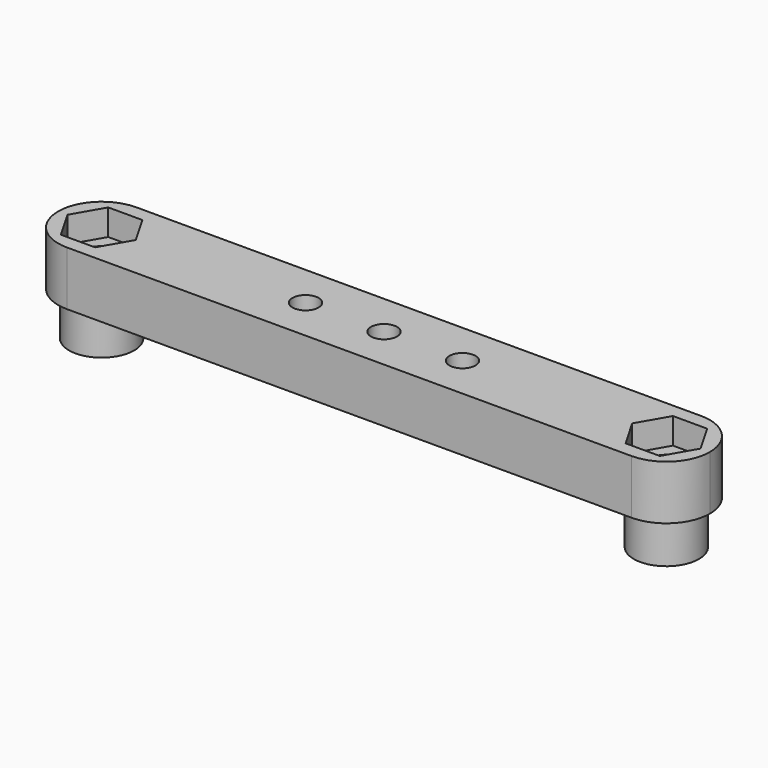
from build123d import *

# Parameters (mm, degrees)
F2_W      = 60
F2_H      = 8
F2_R      = 3
F5_DEPTH  = 5
F1_R      = 3
F1_R_2    = 1.7
F6_DEPTH  = 4
F0_R      = 1.7
F7_DEPTH  = 12.5
F3_R      = 2.05
F8_DEPTH  = 2
F9_DEPTH  = 2
F11_DEPTH = 2.4
F12_R     = 3.99999
F4_R      = 1.2
F13_DEPTH = 5.001


# Not quite as in the source:
# - a fillet or chamfer is up to 0.001 mm smaller than in the source, because OpenCascade refuses the exact size


with BuildPart() as f5:
    # F2 (on face) → F5 (new body)
    with BuildSketch(Plane.XY):
        with Locations((0, 38)):
            Rectangle(F2_W, F2_H)
        with Locations((-26, 38)):
            Circle(F2_R, mode=Mode.SUBTRACT)
        Polygon((1.1402667816, 36.025), (0, 36.025), (-1.1402667816, 36.025), (-2.2805335633, 38), (-1.1402667816, 39.975), (0, 39.975), (1.1402667816, 39.975), (2.2805335633, 38), align=None, mode=Mode.SUBTRACT)
        with Locations((26, 38)):
            Circle(F2_R, mode=Mode.SUBTRACT)
        Polygon((-1.1402667816, 36.025), (0, 36.025), (1.1402667816, 36.025), (2.2805335633, 38), (1.1402667816, 39.975), (0, 39.975), (-1.1402667816, 39.975), (-2.2805335633, 38), align=None)
        with Locations((-26, 38)):
            Circle(F2_R)
        with Locations((26, 38)):
            Circle(F2_R)
    extrude(amount=F5_DEPTH)

    # F1 (on Top) → F6 (join)
    with BuildSketch(Plane.XY):
        with Locations((-26, 38)):
            Circle(F1_R)
        with Locations((-26, 38)):
            Circle(F1_R_2, mode=Mode.SUBTRACT)
        with Locations((26, 38)):
            Circle(F1_R)
        with Locations((26, 38)):
            Circle(F1_R_2, mode=Mode.SUBTRACT)
    extrude(amount=-F6_DEPTH)

    # F0 (on Top) → F7 (cut, symmetric)
    with BuildSketch(Plane.XY):
        with Locations((-26, 38)):
            Circle(F0_R)
        with Locations((26, 38)):
            Circle(F0_R)
        with Locations((-26, -38)):
            Circle(F0_R)
        with Locations((26, -38)):
            Circle(F0_R)
    extrude(amount=F7_DEPTH, both=True, mode=Mode.SUBTRACT)

    # F3 (on face) → F8 (cut)
    with BuildSketch(Plane.XY):
        with Locations((-7.225, 38)):
            Circle(F3_R)
        with Locations((7.225, 38)):
            Circle(F3_R)
    extrude(amount=F8_DEPTH, mode=Mode.SUBTRACT)

    # F2 (on face) → F9 (cut)
    with BuildSketch(Plane.XY):
        Polygon((-1.1402667816, 36.025), (0, 36.025), (1.1402667816, 36.025), (2.2805335633, 38), (1.1402667816, 39.975), (0, 39.975), (-1.1402667816, 39.975), (-2.2805335633, 38), align=None)
    extrude(amount=F9_DEPTH, mode=Mode.SUBTRACT)

    # F10 (on face) → F11 (cut)
    with BuildSketch(Plane.XY.offset(5)):
        Polygon((-27.5732794835, 35.275), (-26, 35.275), (-24.4267205165, 35.275), (-22.8534410329, 38), (-24.4267205165, 40.725), (-26, 40.725), (-27.5732794835, 40.725), (-29.1465589671, 38), align=None)
        Polygon((22.8534410329, 38), (24.4267205165, 35.275), (26, 35.275), (27.5732794835, 35.275), (29.1465589671, 38), (27.5732794835, 40.725), (26, 40.725), (24.4267205165, 40.725), align=None)
    extrude(amount=-F11_DEPTH, mode=Mode.SUBTRACT)

    # F12 (radius 4 in the source; OpenCascade refuses exactly that, so slightly less here)
    f12_edges = [f5.edges().sort_by_distance(p)[0] for p in [
        (-30, 42, 2.5),
        (-30, 34, 2.5),
        (30, 42, 2.5),
        (30, 34, 2.5),
    ]]
    fillet(f12_edges, radius=F12_R)

    # F4 (on face) → F13 (cut, through all)
    with BuildSketch(Plane.XY):
        with Locations((-7.225, 38)):
            Circle(F4_R)
        with Locations((0, 38)):
            Circle(F4_R)
        with Locations((7.225, 38)):
            Circle(F4_R)
    extrude(amount=F13_DEPTH, mode=Mode.SUBTRACT)


solid = f5.part
